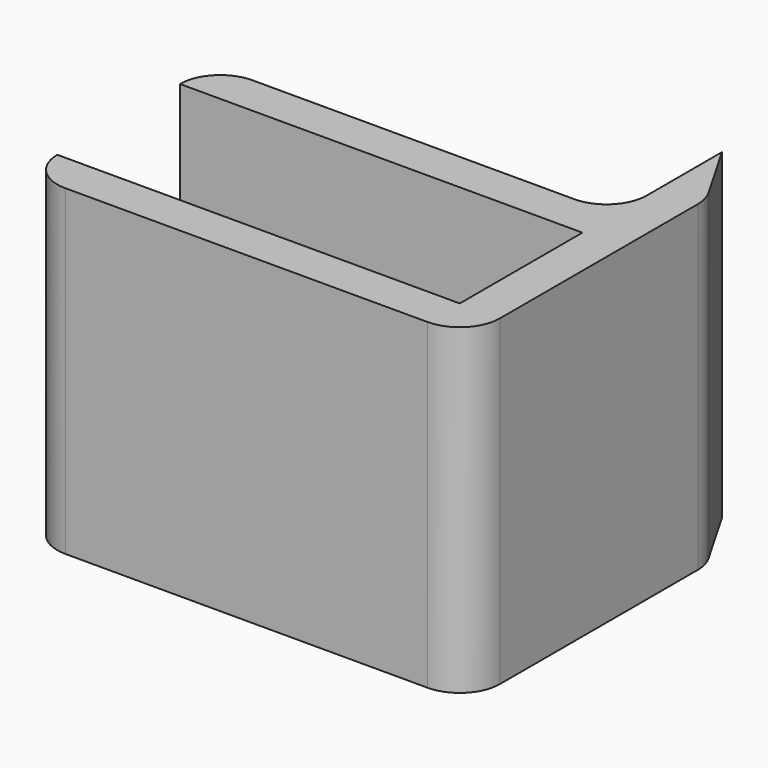
from build123d import *

# Parameters (mm, degrees)
F1_DEPTH = 40
F2_R     = 4.99999


# Not quite as in the source:
# - a fillet or chamfer is up to 0.001 mm smaller than in the source, because OpenCascade refuses the exact size


with BuildPart() as f1:
    # F0 (on Top) → F1 (new body)
    with BuildSketch(Plane.XY):
        Polygon((-27.5, -14.525), (27.5, -14.525), (27.5, 14.525), (27.5, 22.525), (22.5, 31.1852540378), (22.5, 22.525), (22.5, 14.525), (-27.5, 14.525), (-27.5, 9.525), (22.5, 9.525), (22.5, -9.525), (-27.5, -9.525), align=None)
    extrude(amount=F1_DEPTH)

    # F2 (radius 5 in the source; OpenCascade refuses exactly that, so slightly less here)
    f2_edges = [f1.edges().sort_by_distance(p)[0] for p in [
        (-27.5, 14.525, 20),
        (-27.5, -14.525, 20),
        (27.5, -14.525, 20),
        (27.5, 22.525, 20),
        (22.5, 14.525, 20),
    ]]
    fillet(f2_edges, radius=F2_R)


solid = f1.part
